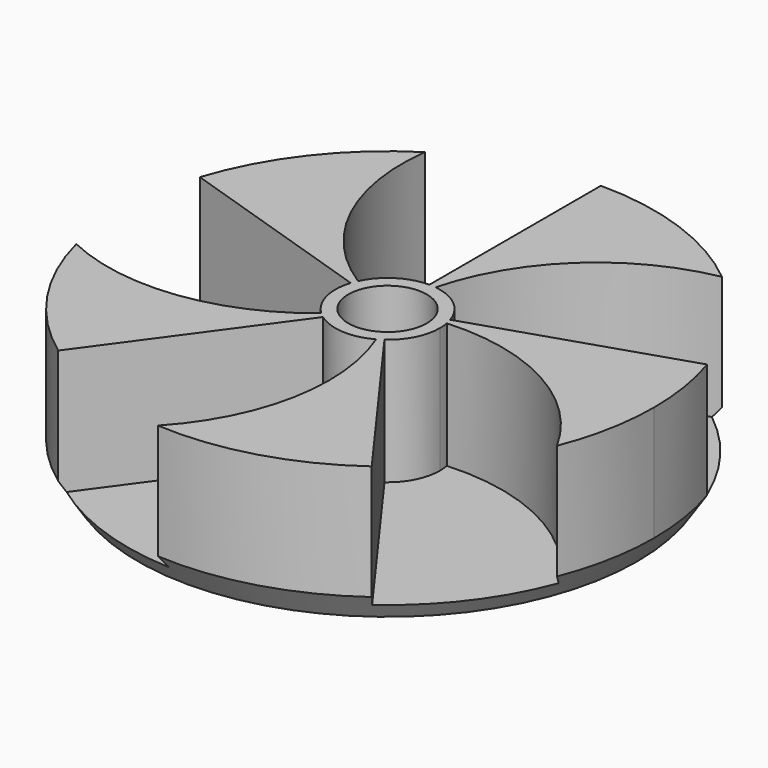
from build123d import *

# Parameters (mm, degrees)
F0_R     = 51
F1_DEPTH = 3
F3_DEPTH = 24
F5_DEPTH = 3
F6_R     = 1.6
F7_DEPTH = 24.001
F8_R     = 7.5
F9_DEPTH = 8


# Not quite as in the source:
# - a fillet or chamfer that OpenCascade refuses, or shapes differently, is made with other operations: its cross-section is extruded or revolved along the edge and cut away or added


with BuildPart() as f1:
    # F0 (on Top) → F1 (new body)
    with BuildSketch(Plane.XY):
        Circle(F0_R)
    extrude(amount=F1_DEPTH)

    # F2 (on face) → F3 (join)
    with BuildSketch(Plane.XY.offset(3)):
        with BuildLine():
            Line((0, 51), (0, 10))
            ThreePointArc((0, 10), (0.6262291254, 9.9803725924), (1.25, 9.9215674165))
            ThreePointArc((1.25, 9.9215674165), (12.6111994349, 29.1522486886), (32.5125, 39.2929681209))
            ThreePointArc((32.5125, 39.2929681209), (17.2780008368, 47.9840670127), (0, 51))
        make_face()
        with BuildLine():
            Line((48.5038823311, 15.7598667131), (9.510565163, 3.0901699437))
            ThreePointArc((9.510565163, 3.0901699437), (9.6854138312, 2.4885254508), (9.8222425863, 1.8771122972))
            ThreePointArc((9.8222425863, 1.8771122972), (31.6225110248, -2.9854231318), (47.4167484056, -18.7790300773))
            ThreePointArc((47.4167484056, -18.7790300773), (50.0961783407, -9.5589181217), (51, 0))
            ThreePointArc((51, 0), (50.3721053704, 7.9781577171), (48.5038823311, 15.7598667131))
        make_face()
        with BuildLine():
            Line((29.9770478669, -41.2598667131), (5.8778525229, -8.0901699437))
            ThreePointArc((5.8778525229, -8.0901699437), (5.3596858173, -8.4423792819), (4.8204797641, -8.7614482161))
            ThreePointArc((4.8204797641, -8.7614482161), (6.9325871881, -30.9973416549), (-3.2073378494, -50.8990469844))
            ThreePointArc((-3.2073378494, -50.8990469844), (14.2261306293, -48.9756797535), (29.9770478669, -41.2598667131))
        make_face()
        with BuildLine():
            Line((-29.9770478669, -41.2598667131), (-5.8778525229, -8.0901699437))
            ThreePointArc((-5.8778525229, -8.0901699437), (-6.372945827, -7.7062027929), (-6.84302225, -7.2919850854))
            ThreePointArc((-6.84302225, -7.2919850854), (-27.3379365126, -16.1719875718), (-49.3989922099, -12.6783109541))
            ThreePointArc((-49.3989922099, -12.6783109541), (-42.1825232409, -28.6641715916), (-29.9770478669, -41.2598667131))
        make_face()
        with BuildLine():
            Line((-48.5038823311, 15.7598667131), (-9.510565163, 3.0901699437))
            ThreePointArc((-9.510565163, 3.0901699437), (-9.2983829469, 3.6796840317), (-9.0497001003, 4.2547535879))
            ThreePointArc((-9.0497001003, 4.2547535879), (-23.8283611351, 21.0025036698), (-27.3229183463, 43.0634198948))
            ThreePointArc((-27.3229183463, 43.0634198948), (-40.2963637234, 31.2602474506), (-48.5038823311, 15.7598667131))
        make_face()
        with BuildLine():
            ThreePointArc((-9.0497001003, 4.2547535879), (-4.6583345766, 1.8434602504), (0, 0))
            Line((0, 0), (0, 10))
            ThreePointArc((0, 10), (-5.3596858173, 8.4423792819), (-9.0497001003, 4.2547535879))
        make_face()
        with BuildLine():
            Line((-9.510565163, 3.0901699437), (0, 0))
            ThreePointArc((0, 0), (-4.6583345766, 1.8434602504), (-9.0497001003, 4.2547535879))
            ThreePointArc((-9.0497001003, 4.2547535879), (-9.2983829469, 3.6796840317), (-9.510565163, 3.0901699437))
        make_face()
        with BuildLine():
            ThreePointArc((-6.84302225, -7.2919850854), (-3.1927394333, -3.8606789083), (0, 0))
            Line((0, 0), (-9.510565163, 3.0901699437))
            ThreePointArc((-9.510565163, 3.0901699437), (-9.6854138312, -2.4885254508), (-6.84302225, -7.2919850854))
        make_face()
        with BuildLine():
            ThreePointArc((4.8204797641, -8.7614482161), (2.6851130896, -4.2294910354), (0, 0))
            Line((0, 0), (-5.8778525229, -8.0901699437))
            ThreePointArc((-5.8778525229, -8.0901699437), (-0.6262291254, -9.9803725924), (4.8204797641, -8.7614482161))
        make_face()
        with BuildLine():
            Line((-5.8778525229, -8.0901699437), (0, 0))
            ThreePointArc((0, 0), (-3.1927394333, -3.8606789083), (-6.84302225, -7.2919850854))
            ThreePointArc((-6.84302225, -7.2919850854), (-6.372945827, -7.7062027929), (-5.8778525229, -8.0901699437))
        make_face()
        with BuildLine():
            Line((5.8778525229, -8.0901699437), (0, 0))
            ThreePointArc((0, 0), (2.6851130896, -4.2294910354), (4.8204797641, -8.7614482161))
            ThreePointArc((4.8204797641, -8.7614482161), (5.3596858173, -8.4423792819), (5.8778525229, -8.0901699437))
        make_face()
        with BuildLine():
            ThreePointArc((9.8222425863, 1.8771122972), (4.8522305863, 1.2467096933), (0, 0))
            Line((0, 0), (5.8778525229, -8.0901699437))
            ThreePointArc((5.8778525229, -8.0901699437), (8.9100652419, -4.5399049974), (10, 0))
            ThreePointArc((10, 0), (9.9554614625, 0.9427550417), (9.8222425863, 1.8771122972))
        make_face()
        with BuildLine():
            Line((9.510565163, 3.0901699437), (0, 0))
            ThreePointArc((0, 0), (4.8522305863, 1.2467096933), (9.8222425863, 1.8771122972))
            ThreePointArc((9.8222425863, 1.8771122972), (9.6854138312, 2.4885254508), (9.510565163, 3.0901699437))
        make_face()
        with BuildLine():
            ThreePointArc((1.25, 9.9215674165), (0.313730334, 5), (0, 0))
            Line((0, 0), (9.510565163, 3.0901699437))
            ThreePointArc((9.510565163, 3.0901699437), (6.372945827, 7.7062027929), (1.25, 9.9215674165))
        make_face()
        with BuildLine():
            Line((0, 10), (0, 0))
            ThreePointArc((0, 0), (0.313730334, 5), (1.25, 9.9215674165))
            ThreePointArc((1.25, 9.9215674165), (0.6262291254, 9.9803725924), (0, 10))
        make_face()
    extrude(amount=F3_DEPTH)

    # F4 (on face) → F5 (cut)
    with BuildSketch(Plane(origin=(0, 0, 0), x_dir=(1, 0, 0), z_dir=(0, 0, -1))):
        Polygon((2.75, -1.5877132403), (2.75, 1.5877132403), (0, 3.1754264805), (-2.75, 1.5877132403), (-2.75, -1.5877132403), (0, -3.1754264805), align=None)
    extrude(amount=-F5_DEPTH, mode=Mode.SUBTRACT)

    # F6 (on face) → F7 (cut, through all)
    with BuildSketch(Plane(origin=(0, 0, 3), x_dir=(1, 0, 0), z_dir=(0, 0, -1))):
        Circle(F6_R)
    extrude(amount=-F7_DEPTH, mode=Mode.SUBTRACT)

    # F8 (on face) → F9 (cut)
    with BuildSketch(Plane.XY.offset(27)):
        Circle(F8_R)
    extrude(amount=-F9_DEPTH, mode=Mode.SUBTRACT)

    # F10: chamfer of 5 x 3.247037966 on 1 edges, made by hand

    # F10_s1 → F10_t2 (revolve, cut)
    with BuildSketch(Plane.XZ):
        Polygon((51, 5), (47.752962034, 0), (51, 0), align=None)
    revolve(axis=Axis((0, 0, 0), (0, 0, 1)), mode=Mode.SUBTRACT)


solid = f1.part
